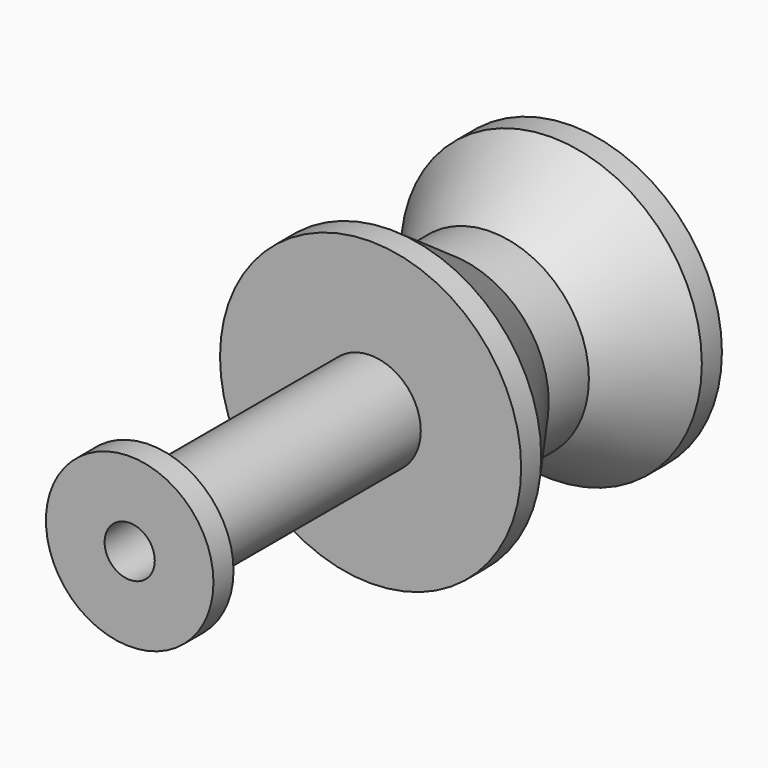
from build123d import *

# Parameters (mm, degrees)
F0_R      = 2
F0_R_2    = 1
F1_DEPTH  = 22
F0_R_3    = 6
F0_R_4    = 3.5
F2_DEPTH  = 1
F2_FACE_R = 6
F3_DEPTH  = 3
F3_TAPER  = 35
F4_DEPTH  = 2
F7_R      = 3.33782825
F7_R_2    = 2
F7_R_3    = 1
F8_DEPTH  = 1


# Not quite as in the source:
# - a feature of the source that left no trace in its solid (it failed there, or was rolled back) is left out
# - a pattern or mirror of a feature is missing from the dataset's text; its kind, count and spacing are read off the source's solid


with BuildPart() as f1:
    # F0 (on Front) → F1 (new body)
    with BuildSketch(Plane.XZ):
        Circle(F0_R)
        Circle(F0_R_2, mode=Mode.SUBTRACT)
    extrude(amount=F1_DEPTH)

    # F2_copies: F2 across plane


with BuildPart() as f2:
    # F0 (on Front) → F2 (new body)
    with BuildSketch(Plane.XZ):
        Circle(F0_R_3)
        Circle(F0_R_4, mode=Mode.SUBTRACT)
        Circle(F0_R_4)
        Circle(F0_R, mode=Mode.SUBTRACT)
        Circle(F0_R)
        Circle(F0_R_2, mode=Mode.SUBTRACT)
        Circle(F0_R_2)
    extrude(amount=F2_DEPTH)


with BuildPart() as f1_1:
    add(f1.part)
    add(f2.part.mirror(Plane(origin=(0, -5, 0), x_dir=(0, 0, -1), z_dir=(0, -1, 0))))


    add(f2.part)  # F3 merges F2
    # F2_face (on face) → F3 (join)
    with BuildSketch(Plane.XZ.offset(1)):
        Circle(F2_FACE_R)
    f3 = extrude(amount=F3_DEPTH, taper=F3_TAPER)

    # F3_copies: F3 across plane
    add(f3.mirror(Plane(origin=(0, -5, 0), x_dir=(0, 0, -1), z_dir=(0, -1, 0))))

    # F4 (add): faces of the model
    f4_faces = [f1_1.faces().sort_by_distance(p)[0] for p in [
        (-3.7890863377, -4, 0),
        (0, -4, 0),
    ]]
    extrude(f4_faces, amount=F4_DEPTH)

    # F7 (on face) → F8 (join)
    with BuildSketch(Plane.XZ.offset(22)):
        Circle(F7_R)
        Circle(F7_R_2, mode=Mode.SUBTRACT)
        Circle(F7_R_2)
        Circle(F7_R_3, mode=Mode.SUBTRACT)
    extrude(amount=-F8_DEPTH)


solid = f1_1.part
